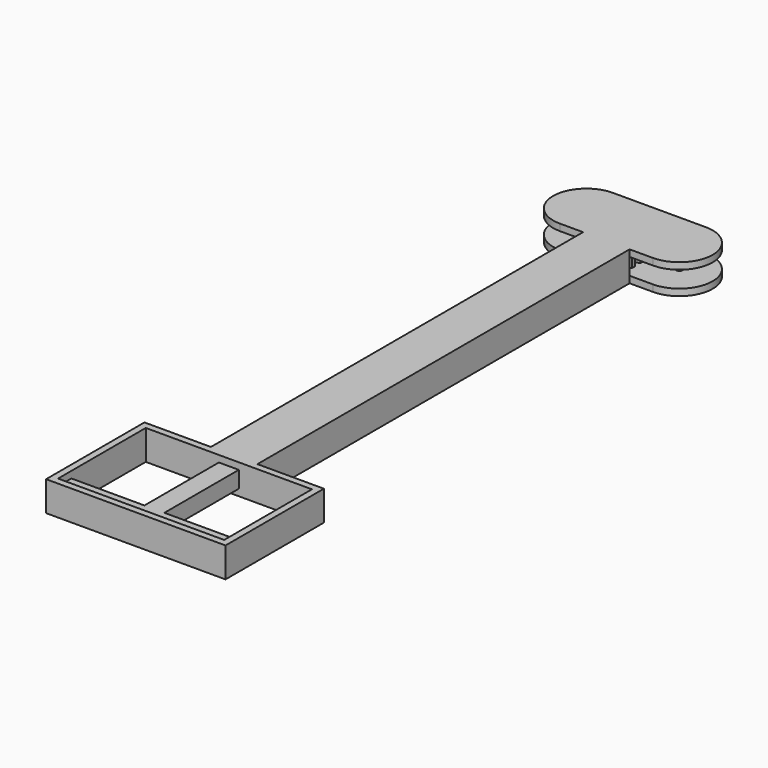
from build123d import *

# Parameters (mm, degrees)
F1_DEPTH      = 5
F3_W          = 50
F3_H          = 5
F4_DEPTH      = 5
F5_W          = 50
F5_H          = 33
F6_DEPTH      = 7
F6_DEPTH_BACK = 2
F9_DEPTH      = 5
F10_W         = 10
F10_H         = 5
F11_DEPTH     = 50
F12_R         = 1
F13_DEPTH     = 5


with BuildPart() as f1:
    # F0 (on Top) → F1 (new body)
    with BuildSketch(Plane.XY):
        Polygon((0, 13), (0, -180), (3, -180), (3, -39.0871235167), (3, -36.9128764833), (3, -35.8871235167), (3, -33.7128764833), (3, -32.6871235167), (3, -30.5128764833), (3, -29.4871235167), (3, -27.3128764833), (3, -26.2871235167), (3, -24.1128764833), (3, -23.0871235167), (3, -20.9128764833), (3, -19.8871235167), (3, -17.7128764833), (3, -16.6871235167), (3, -14.5128764833), (3, -13.4871235167), (3, -11.3128764833), (3, -10.2871235167), (3, -8.1128764833), (3, -7.0871235167), (3, -4.9128764833), (3, -3.8871235167), (3, -1.7128764833), (3, -0.6871235167), (3, 1.4871235167), (3, 2.5128764833), (3, 4.6871235167), (3, 5.7128764833), (3, 7.8871235167), (3, 8.9128764833), (3, 11.0871235167), (3, 13), align=None)
        with BuildLine():
            Line((3, -36.9128764833), (3, -39.0871235167))
            ThreePointArc((3, -39.0871235167), (4.0421988802, -38.9373096378), (5, -38.5))
            Line((5, -38.5), (5, -38))
            Line((5, -38), (5, -37.5))
            ThreePointArc((5, -37.5), (4.0421988802, -37.0626903622), (3, -36.9128764833))
        make_face()
        with BuildLine():
            ThreePointArc((5, 10.5), (4.0421988802, 10.9373096378), (3, 11.0871235167))
            Line((3, 11.0871235167), (3, 8.9128764833))
            ThreePointArc((3, 8.9128764833), (4.0421988802, 9.0626903622), (5, 9.5))
            Line((5, 9.5), (5, 10))
            Line((5, 10), (5, 10.5))
        make_face()
        with BuildLine():
            Line((3, -33.7128764833), (3, -35.8871235167))
            ThreePointArc((3, -35.8871235167), (4.0421988802, -35.7373096378), (5, -35.3))
            Line((5, -35.3), (5, -34.8))
            Line((5, -34.8), (5, -34.3))
            ThreePointArc((5, -34.3), (4.0421988802, -33.8626903622), (3, -33.7128764833))
        make_face()
        with BuildLine():
            ThreePointArc((5, 7.3), (4.0421988802, 7.7373096378), (3, 7.8871235167))
            Line((3, 7.8871235167), (3, 5.7128764833))
            ThreePointArc((3, 5.7128764833), (4.0421988802, 5.8626903622), (5, 6.3))
            Line((5, 6.3), (5, 6.8))
            Line((5, 6.8), (5, 7.3))
        make_face()
        with BuildLine():
            Line((3, -30.5128764833), (3, -32.6871235167))
            ThreePointArc((3, -32.6871235167), (4.0421988802, -32.5373096378), (5, -32.1))
            Line((5, -32.1), (5, -31.6))
            Line((5, -31.6), (5, -31.1))
            ThreePointArc((5, -31.1), (4.0421988802, -30.6626903622), (3, -30.5128764833))
        make_face()
        with BuildLine():
            ThreePointArc((5, 4.1), (4.0421988802, 4.5373096378), (3, 4.6871235167))
            Line((3, 4.6871235167), (3, 2.5128764833))
            ThreePointArc((3, 2.5128764833), (4.0421988802, 2.6626903622), (5, 3.1))
            Line((5, 3.1), (5, 3.6))
            Line((5, 3.6), (5, 4.1))
        make_face()
        with BuildLine():
            Line((3, -27.3128764833), (3, -29.4871235167))
            ThreePointArc((3, -29.4871235167), (4.0421988802, -29.3373096378), (5, -28.9))
            Line((5, -28.9), (5, -28.4))
            Line((5, -28.4), (5, -27.9))
            ThreePointArc((5, -27.9), (4.0421988802, -27.4626903622), (3, -27.3128764833))
        make_face()
        with BuildLine():
            ThreePointArc((5, 0.9), (4.0421988802, 1.3373096378), (3, 1.4871235167))
            Line((3, 1.4871235167), (3, -0.6871235167))
            ThreePointArc((3, -0.6871235167), (4.0421988802, -0.5373096378), (5, -0.1))
            Line((5, -0.1), (5, 0.4))
            Line((5, 0.4), (5, 0.9))
        make_face()
        with BuildLine():
            Line((3, -24.1128764833), (3, -26.2871235167))
            ThreePointArc((3, -26.2871235167), (4.0421988802, -26.1373096378), (5, -25.7))
            Line((5, -25.7), (5, -25.2))
            Line((5, -25.2), (5, -24.7))
            ThreePointArc((5, -24.7), (4.0421988802, -24.2626903622), (3, -24.1128764833))
        make_face()
        with BuildLine():
            ThreePointArc((5, -2.3), (4.0421988802, -1.8626903622), (3, -1.7128764833))
            Line((3, -1.7128764833), (3, -3.8871235167))
            ThreePointArc((3, -3.8871235167), (4.0421988802, -3.7373096378), (5, -3.3))
            Line((5, -3.3), (5, -2.8))
            Line((5, -2.8), (5, -2.3))
        make_face()
        with BuildLine():
            Line((3, -20.9128764833), (3, -23.0871235167))
            ThreePointArc((3, -23.0871235167), (4.0421988802, -22.9373096378), (5, -22.5))
            Line((5, -22.5), (5, -22))
            Line((5, -22), (5, -21.5))
            ThreePointArc((5, -21.5), (4.0421988802, -21.0626903622), (3, -20.9128764833))
        make_face()
        with BuildLine():
            ThreePointArc((5, -5.5), (4.0421988802, -5.0626903622), (3, -4.9128764833))
            Line((3, -4.9128764833), (3, -7.0871235167))
            ThreePointArc((3, -7.0871235167), (4.0421988802, -6.9373096378), (5, -6.5))
            Line((5, -6.5), (5, -6))
            Line((5, -6), (5, -5.5))
        make_face()
        with BuildLine():
            Line((3, -17.7128764833), (3, -19.8871235167))
            ThreePointArc((3, -19.8871235167), (4.0421988802, -19.7373096378), (5, -19.3))
            Line((5, -19.3), (5, -18.8))
            Line((5, -18.8), (5, -18.3))
            ThreePointArc((5, -18.3), (4.0421988802, -17.8626903622), (3, -17.7128764833))
        make_face()
        with BuildLine():
            ThreePointArc((5, -8.7), (4.0421988802, -8.2626903622), (3, -8.1128764833))
            Line((3, -8.1128764833), (3, -10.2871235167))
            ThreePointArc((3, -10.2871235167), (4.0421988802, -10.1373096378), (5, -9.7))
            Line((5, -9.7), (5, -9.2))
            Line((5, -9.2), (5, -8.7))
        make_face()
        with BuildLine():
            Line((3, -14.5128764833), (3, -16.6871235167))
            ThreePointArc((3, -16.6871235167), (4.0421988802, -16.5373096378), (5, -16.1))
            Line((5, -16.1), (5, -15.6))
            Line((5, -15.6), (5, -15.1))
            ThreePointArc((5, -15.1), (4.0421988802, -14.6626903622), (3, -14.5128764833))
        make_face()
        with BuildLine():
            ThreePointArc((5, -11.9), (4.0421988802, -11.4626903622), (3, -11.3128764833))
            Line((3, -11.3128764833), (3, -13.4871235167))
            ThreePointArc((3, -13.4871235167), (4.0421988802, -13.3373096378), (5, -12.9))
            Line((5, -12.9), (5, -12.4))
            Line((5, -12.4), (5, -11.9))
        make_face()
    extrude(amount=F1_DEPTH)

    # F2: F1 across face


with BuildPart() as f1_1:
    add(f1.part)
    add(f1.part.mirror(Plane(origin=(0, -83.5, 2.5), x_dir=(0, -1, 0), z_dir=(-1, 0, 0))))

    # F3 (on face) → F4 (join)
    with BuildSketch(Plane.XZ.offset(180)):
        with Locations((0, 2.5)):
            Rectangle(F3_W, F3_H)
    extrude(amount=F4_DEPTH)


with BuildPart() as f6:
    # F5 (on Top) → F6 (new body, two sides)
    with BuildSketch(Plane.XY) as f6_sk:
        with BuildLine():
            ThreePointArc((14, -10), (21.0710678119, -7.0710678119), (24, 0))
            ThreePointArc((24, 0), (21.0710678119, 7.0710678119), (14, 10))
            ThreePointArc((14, 10), (4, 0), (14, -10))
        make_face()
        with BuildLine():
            ThreePointArc((14, -10), (4, 0), (14, 10))
            Line((14, 10), (0, 10))
            Line((0, 10), (-14, 10))
            ThreePointArc((-14, 10), (-6.9289321881, 7.0710678119), (-4, 0))
            ThreePointArc((-4, 0), (-6.9289321881, -7.0710678119), (-14, -10))
            Line((-14, -10), (-7, -10))
            Line((-7, -10), (-7, -150))
            Line((-7, -150), (-27, -150))
            Line((-27, -150), (-27, -187))
            Line((-27, -187), (0, -187))
            Line((0, -187), (27, -187))
            Line((27, -187), (27, -150))
            Line((27, -150), (7, -150))
            Line((7, -150), (7, -10))
            Line((7, -10), (14, -10))
        make_face()
        with Locations((0, -168.5)):
            Rectangle(F5_W, F5_H, mode=Mode.SUBTRACT)
        with BuildLine():
            ThreePointArc((-4, 0), (-6.9289321881, 7.0710678119), (-14, 10))
            ThreePointArc((-14, 10), (-24, 0), (-14, -10))
            ThreePointArc((-14, -10), (-6.9289321881, -7.0710678119), (-4, 0))
        make_face()
    extrude(amount=F6_DEPTH)
    extrude(f6_sk.sketch, amount=-F6_DEPTH_BACK)

    # F7: cut F1
    add(f1_1.part, mode=Mode.SUBTRACT)

    # F8 (on Top) → F9 (cut)
    with BuildSketch(Plane.XY):
        with BuildLine():
            ThreePointArc((-14, 10), (-24, 0), (-14, -10))
            Line((-14, -10), (14, -10))
            ThreePointArc((14, -10), (24, 0), (14, 10))
            Line((14, 10), (-14, 10))
        make_face()
    extrude(amount=F9_DEPTH, mode=Mode.SUBTRACT)

    # F10 (on face) → F11 (cut)
    with BuildSketch(Plane(origin=(0, -10, 0), x_dir=(-1, 0, 0), z_dir=(0, 1, 0))):
        with Locations((0, 2.5)):
            Rectangle(F10_W, F10_H)
    extrude(amount=-F11_DEPTH, mode=Mode.SUBTRACT)

    # F12 (on face) → F13 (join, through all)
    with BuildSketch(Plane.XY):
        with Locations((-14, 0)):
            Circle(F12_R)
        with Locations((14, 0)):
            Circle(F12_R)
    extrude(amount=F13_DEPTH)


solid = Compound([f1_1.part, f6.part])
